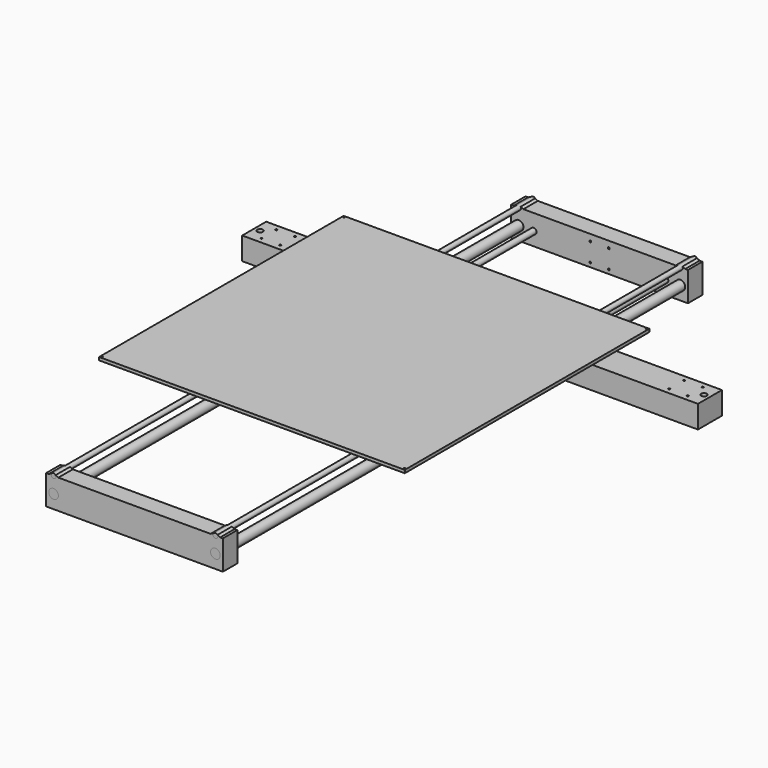
from build123d import *

# Parameters (mm, degrees)
F0_W            = 510
F0_H            = 510
F0_R            = 1.5
F1_DEPTH        = 5
F4_R            = 4
F5_DEPTH        = 500
F6_R            = 8
F7_DEPTH        = 1000
F8_DEPTH        = 30
F9_R            = 8
F9_R_2          = 4.8
F10_DEPTH       = 30
F11_DEPTH       = 300
F12_W           = 290
F12_H           = 50
F13_DEPTH       = 37.75
F14_R           = 4.8
F15_DEPTH       = 25
F18_D           = 3
F18_CSINK_D     = 6
F18_CSINK_ANGLE = 90
F19_D           = 3
F19_CSINK_D     = 6
F19_CSINK_ANGLE = 90


# Not quite as in the source:
# - a feature names something its author has since deleted; it is built from what else it names


with BuildPart() as f1:
    # F0 (on Top) → F1 (new body)
    with BuildSketch(Plane.XY):
        Rectangle(F0_W, F0_H)
        with Locations((-252.5, -252.5)):
            Circle(F0_R, mode=Mode.SUBTRACT)
        with Locations((252.5, -252.5)):
            Circle(F0_R, mode=Mode.SUBTRACT)
        with Locations((-252.5, 252.5)):
            Circle(F0_R, mode=Mode.SUBTRACT)
        with Locations((252.5, 252.5)):
            Circle(F0_R, mode=Mode.SUBTRACT)
    extrude(amount=F1_DEPTH)


with BuildPart() as f5:
    # F4 (on Front) → F5 (new body, symmetric)
    with BuildSketch(Plane.XZ):
        with Locations((-135, -31)):
            Circle(F4_R)
    extrude(amount=F5_DEPTH, both=True)


with BuildPart() as f5b:
    # F4 (on Front) → F5, piece 2 (new body, symmetric)
    with BuildSketch(Plane.XZ):
        with Locations((135, -31)):
            Circle(F4_R)
    extrude(amount=F5_DEPTH, both=True)


with BuildPart() as f7:
    # F6 (on face) → F7 (new body, through all)
    with BuildSketch(Plane.XZ.offset(500)):
        with Locations((135, -57.5)):
            Circle(F6_R)
    extrude(amount=-F7_DEPTH)


with BuildPart() as f7b:
    # F6 (on face) → F7, piece 2 (new body, through all)
    with BuildSketch(Plane.XZ.offset(500)):
        with Locations((-135, -57.5)):
            Circle(F6_R)
    extrude(amount=-F7_DEPTH)


with BuildPart() as f8:
    # F6 (on face) → F8 (new body)
    with BuildSketch(Plane.XZ.offset(500)):
        with BuildLine():
            Line((-127, -31), (-131, -31))
            ThreePointArc((-131, -31), (-135, -35), (-139, -31))
            Line((-139, -31), (-143, -31))
            Line((-143, -31), (-147.5, -31))
            Line((-147.5, -31), (-147.5, -80))
            Line((-147.5, -80), (147.5, -80))
            Line((147.5, -80), (147.5, -31))
            Line((147.5, -31), (143, -31))
            Line((143, -31), (139, -31))
            ThreePointArc((139, -31), (135, -35), (131, -31))
            Line((131, -31), (127, -31))
            Line((127, -31), (-127, -31))
        make_face()
        with Locations((-135, -57.5)):
            Circle(F6_R, mode=Mode.SUBTRACT)
        with Locations((135, -57.5)):
            Circle(F6_R, mode=Mode.SUBTRACT)
        with BuildLine():
            Line((-143, -31), (-139, -31))
            ThreePointArc((-139, -31), (-138.8428168516, -29.8897033527), (-138.3836206775, -28.8666666667))
            ThreePointArc((-138.3836206775, -28.8666666667), (-140.7908965377, -29.7189179521), (-143, -31))
        make_face()
        with BuildLine():
            ThreePointArc((-131.6163793225, -28.8666666667), (-131.1571831484, -29.8897033527), (-131, -31))
            Line((-131, -31), (-127, -31))
            ThreePointArc((-127, -31), (-129.2091034623, -29.7189179521), (-131.6163793225, -28.8666666667))
        make_face()
        with BuildLine():
            ThreePointArc((131.6163793225, -28.8666666667), (129.2091034623, -29.7189179521), (127, -31))
            Line((127, -31), (131, -31))
            ThreePointArc((131, -31), (131.1571831484, -29.8897033527), (131.6163793225, -28.8666666667))
        make_face()
        with BuildLine():
            ThreePointArc((138.3836206775, -28.8666666667), (138.8428168516, -29.8897033527), (139, -31))
            Line((139, -31), (143, -31))
            ThreePointArc((143, -31), (140.7908965377, -29.7189179521), (138.3836206775, -28.8666666667))
        make_face()
    extrude(amount=-F8_DEPTH)


with BuildPart() as f10:
    # F9 (on face) → F10 (new body)
    with BuildSketch(Plane(origin=(0, 500, 0), x_dir=(-1, 0, 0), z_dir=(0, 1, 0))):
        with BuildLine():
            ThreePointArc((-131.6163793225, -28.8666666667), (-135, -35), (-138.3836206775, -28.8666666667))
            ThreePointArc((-138.3836206775, -28.8666666667), (-140.7908965377, -29.7189179521), (-143, -31))
            Line((-143, -31), (-147.5, -31))
            Line((-147.5, -31), (-147.5, -80))
            Line((-147.5, -80), (147.5, -80))
            Line((147.5, -80), (147.5, -31))
            Line((147.5, -31), (143, -31))
            ThreePointArc((143, -31), (140.7908965377, -29.7189179521), (138.3836206775, -28.8666666667))
            ThreePointArc((138.3836206775, -28.8666666667), (138.8428168516, -29.8897033527), (139, -31))
            ThreePointArc((139, -31), (133.8897033527, -34.8428168516), (131.6163793225, -28.8666666667))
            ThreePointArc((131.6163793225, -28.8666666667), (129.2091034623, -29.7189179521), (127, -31))
            Line((127, -31), (-127, -31))
            ThreePointArc((-127, -31), (-129.2091034623, -29.7189179521), (-131.6163793225, -28.8666666667))
        make_face()
        with Locations((-135, -57.5)):
            Circle(F9_R, mode=Mode.SUBTRACT)
        with Locations((-110, -57.5)):
            Circle(F9_R_2, mode=Mode.SUBTRACT)
        with Locations((110, -57.5)):
            Circle(F9_R_2, mode=Mode.SUBTRACT)
        with Locations((135, -57.5)):
            Circle(F9_R, mode=Mode.SUBTRACT)
    extrude(amount=-F10_DEPTH)

    # F19 (through all)
    with Locations(Plane(origin=(0, 500, 0), x_dir=(-1, 0, 0), z_dir=(0, 1, 0))):
        with Locations((-15.5, -42), (15.5, -42), (15.5, -73), (-15.5, -73)):
            CounterSinkHole(F19_D / 2, F19_CSINK_D / 2, counter_sink_angle=F19_CSINK_ANGLE)


with BuildPart() as f11:
    # F9 (on face) → F11 (new body)
    with BuildSketch(Plane(origin=(0, 500, 0), x_dir=(-1, 0, 0), z_dir=(0, 1, 0))):
        with Locations((-110, -57.5)):
            Circle(F9_R_2)
    extrude(amount=-F11_DEPTH)


with BuildPart() as f11b:
    # F9 (on face) → F11, piece 2 (new body)
    with BuildSketch(Plane(origin=(0, 500, 0), x_dir=(-1, 0, 0), z_dir=(0, 1, 0))):
        with Locations((110, -57.5)):
            Circle(F9_R_2)
    extrude(amount=-F11_DEPTH)


with BuildPart() as f13:
    # F12 (on face) → F13 (new body, through all)
    with BuildSketch(Plane(origin=(0, 0, -80), x_dir=(1, 0, 0), z_dir=(0, 0, -1))):
        with Locations((-235.2, -225)):
            Rectangle(F12_W, F12_H)
    extrude(amount=-F13_DEPTH)

    # F14 (on face) → F15 (cut)
    with BuildSketch(Plane.XY.offset(-42.25)):
        with Locations((-370.4, 225)):
            Circle(F14_R)
    extrude(amount=-F15_DEPTH, mode=Mode.SUBTRACT)

    # F17: cut F11b, F7b
    add(f11b.part, mode=Mode.SUBTRACT)
    add(f7b.part, mode=Mode.SUBTRACT)

    # F18 (through all)
    with Locations(Plane(origin=(0, 0, -80), x_dir=(1, 0, 0), z_dir=(0, 0, -1))):
        with Locations((-324.6, -240.5), (-355.6, -240.5), (-355.6, -209.5), (-324.6, -209.5)):
            CounterSinkHole(F18_D / 2, F18_CSINK_D / 2, counter_sink_angle=F18_CSINK_ANGLE)


with BuildPart() as f20_1:
    # F20: instance of F13
    add(f13.part.mirror(Plane.YZ))


solid = Compound([f1.part, f5.part, f5b.part, f7.part, f7b.part, f8.part, f10.part, f11.part, f11b.part, f13.part, f20_1.part])
